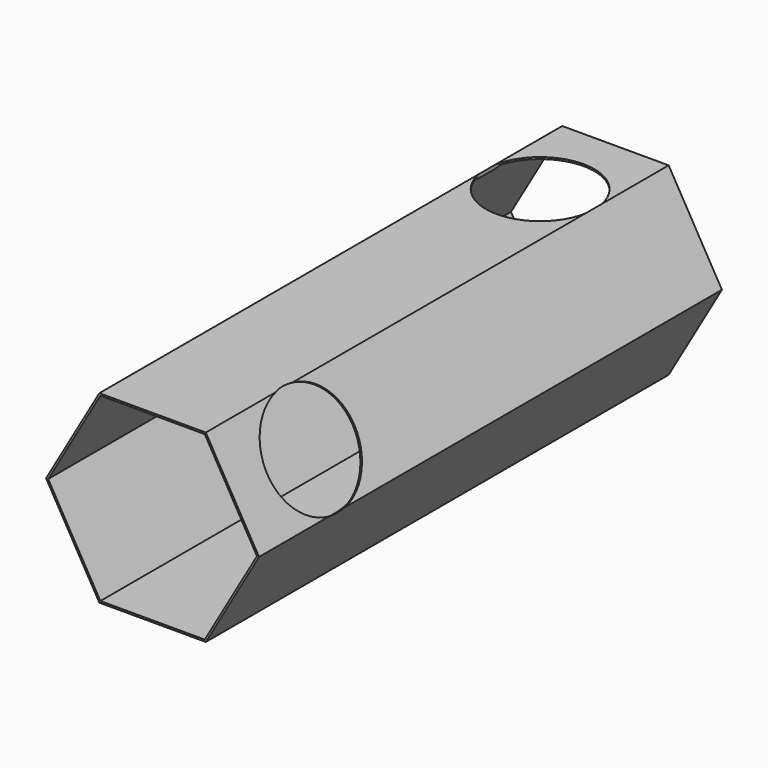
from build123d import *

# Parameters (mm, degrees)
F1_DEPTH = 160
F2_DEPTH = 140
F4_DEPTH = 1.4817621135
F6_DEPTH = 5


# Not quite as in the source:
# - a feature names something its author has since deleted; it is built from what else it names


with BuildPart() as f1:
    # F0 (on Front) → F1 (new body)
    with BuildSketch(Plane.XZ):
        Polygon((14.7224318643, 25.5), (-14.7224318643, 25.5), (-29.4448637287, 0), (-14.7224318643, -25.5), (14.7224318643, -25.5), (29.4448637287, 0), align=None)
        Polygon((-28.8675134595, 0), (-14.4337567297, 25), (14.4337567297, 25), (28.8675134595, 0), (14.4337567297, -25), (12.7224318643, -25), (-12.7224318643, -25), (-14.4337567297, -25), align=None, mode=Mode.SUBTRACT)
    extrude(amount=F1_DEPTH)

    # F0 (on Front) → F2 (join)
    with BuildSketch(Plane.XZ):
        Polygon((14.7224318643, 25.5), (-14.7224318643, 25.5), (-29.4448637287, 0), (-14.7224318643, -25.5), (14.7224318643, -25.5), (29.4448637287, 0), align=None)
        Polygon((-28.8675134595, 0), (-14.4337567297, 25), (14.4337567297, 25), (28.8675134595, 0), (14.4337567297, -25), (12.7224318643, -25), (-12.7224318643, -25), (-14.4337567297, -25), align=None, mode=Mode.SUBTRACT)
    extrude(amount=F2_DEPTH)

    # F3 (on face) → F4 (cut, through all)
    with BuildSketch(Plane(origin=(22.0836477965, 0, 12.75), x_dir=(0, 1, 0), z_dir=(0.8660254038, 0, 0.5))):
        with BuildLine():
            ThreePointArc((-130.0384322302, -14.7224318643), (-121.3330579218, -9.537184599), (-117.9107135534, 0))
            ThreePointArc((-117.9107135534, 0), (-121.3330579218, 9.537184599), (-130.0384322302, 14.7224318643))
            Line((-130.0384322302, 14.7224318643), (-135.7829948767, 14.7224318643))
            ThreePointArc((-135.7829948767, 14.7224318643), (-147.9107135534, 0), (-135.7829948767, -14.7224318643))
            Line((-135.7829948767, -14.7224318643), (-130.0384322302, -14.7224318643))
        make_face()
        with BuildLine():
            ThreePointArc((-135.7829948767, -14.7224318643), (-132.9107135534, -15), (-130.0384322302, -14.7224318643))
            Line((-130.0384322302, -14.7224318643), (-135.7829948767, -14.7224318643))
        make_face()
        with BuildLine():
            Line((-135.7829948767, 14.7224318643), (-130.0384322302, 14.7224318643))
            ThreePointArc((-130.0384322302, 14.7224318643), (-132.9107135534, 15), (-135.7829948767, 14.7224318643))
        make_face()
    extrude(amount=-F4_DEPTH, mode=Mode.SUBTRACT)

    # F5 (on face) → F6 (cut)
    with BuildSketch(Plane.XY.offset(25.5)):
        with BuildLine():
            Line((14.7224318643, -28.900016646), (14.7224318643, -23.1554539994))
            ThreePointArc((14.7224318643, -23.1554539994), (0, -11.0277353227), (-14.7224318643, -23.1554539994))
            Line((-14.7224318643, -23.1554539994), (-14.7224318643, -28.900016646))
            ThreePointArc((-14.7224318643, -28.900016646), (0, -41.0277353227), (14.7224318643, -28.900016646))
        make_face()
    extrude(amount=-F6_DEPTH, mode=Mode.SUBTRACT)


solid = f1.part
